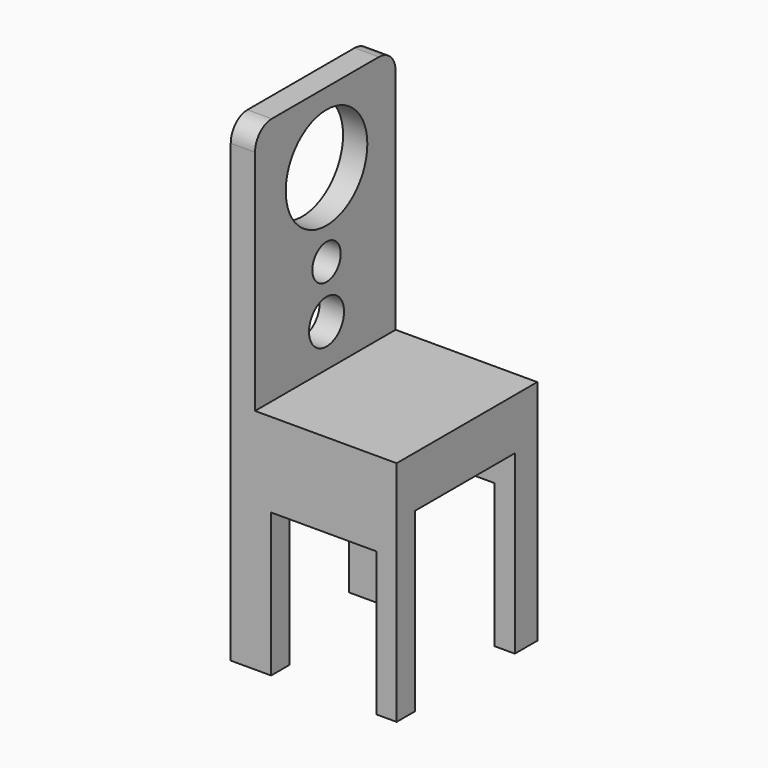
from build123d import *

# Parameters (mm, degrees)
F0_R     = 6.6404165098
F0_R_2   = 5.3780790225
F0_R_3   = 15.463703615
F1_DEPTH = 3.683
F2_W     = 53.2784113497
F2_H     = 69.0371559083
F3_DEPTH = 42.926
F4_W     = 37.8411058336
F4_H     = 53.5067310557
F5_DEPTH = 50.293
F6_W     = 31.9212079048
F6_H     = 43.5216361657
F7_DEPTH = 53.2794113497


# Not quite as in the source:
# - a feature names something its author has since deleted; it is built from what else it names


with BuildPart() as f1:
    # F0 (on Right) → F1 (new body, symmetric)
    with BuildSketch(Plane.YZ):
        with BuildLine():
            Line((19.8416914791, 85.8998820186), (-20.7367198706, 85.8998820186))
            ThreePointArc((-20.7367198706, 85.8998820186), (-25.2268479311, 84.0400100791), (-27.0867198706, 79.5498820186))
            Line((-27.0867198706, 79.5498820186), (-27.0867198706, -58.5244297981))
            Line((-27.0867198706, -58.5244297981), (26.1916914791, -58.5244297981))
            Line((26.1916914791, -58.5244297981), (26.1916914791, 79.5498820186))
            ThreePointArc((26.1916914791, 79.5498820186), (24.3318195396, 84.0400100791), (19.8416914791, 85.8998820186))
        make_face()
        with Locations((0, 23.3183521777)):
            Circle(F0_R, mode=Mode.SUBTRACT)
        with Locations((0, 39.2750576138)):
            Circle(F0_R_2, mode=Mode.SUBTRACT)
        with Locations((0, 64.4399300218)):
            Circle(F0_R_3, mode=Mode.SUBTRACT)
    extrude(amount=F1_DEPTH, both=True)

    # F2 (on face) → F3 (join)
    with BuildSketch(Plane.YZ.offset(3.683)):
        with Locations((-0.4475141957, -24.005851844)):
            Rectangle(F2_W, F2_H)
    extrude(amount=F3_DEPTH)

    # F4 (on face) → F5 (cut, through all)
    with BuildSketch(Plane.YZ.offset(46.609)):
        with Locations((-1.2208549306, -31.7710642703)):
            Rectangle(F4_W, F4_H)
    extrude(amount=-F5_DEPTH, mode=Mode.SUBTRACT)

    # F6 (on face) → F7 (cut, through all)
    with BuildSketch(Plane(origin=(0, 26.1916914791, 0), x_dir=(-1, 0, 0), z_dir=(0, 1, 0))):
        with Locations((-24.5076268911, -36.7636117153)):
            Rectangle(F6_W, F6_H)
    extrude(amount=-F7_DEPTH, mode=Mode.SUBTRACT)


solid = f1.part
